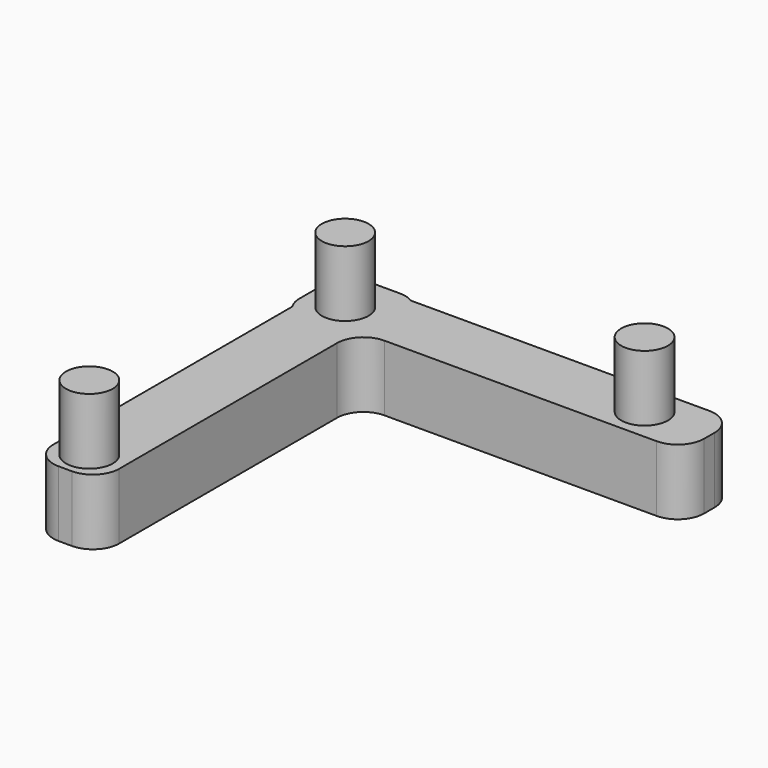
from build123d import *

# Parameters (mm, degrees)
F0_R         = 4.5120624022
F1_DEPTH     = 25.4
F0_W         = 0.7937453203
F0_H         = 12.7
F0_W_2       = 12.7
F0_H_2       = 0.7937453203
F2_DEPTH     = 12.7
F3_R         = 5.08
F4_T1_DEPTH  = 12.7
F4_T3_DEPTH  = 26.333067172
F4_T5_DEPTH  = 38.1
F4_T7_DEPTH  = 26.333067172
F4_T9_DEPTH  = 38.1
F4_T11_DEPTH = 26.333067172
F4_T13_DEPTH = 38.1
F4_T15_DEPTH = 26.333067172


# Not quite as in the source:
# - a fillet or chamfer that OpenCascade refuses, or shapes differently, is made with other operations: its cross-section is extruded or revolved along the edge and cut away or added


with BuildPart() as f1:
    # F0 (on Top) → F1 (new body)
    with BuildSketch(Plane.XY):
        with Locations((-30.9562546797, 29.4322539121)):
            Circle(F0_R)
    extrude(amount=F1_DEPTH)


with BuildPart() as f1b:
    # F0 (on Top) → F1, piece 2 (new body)
    with BuildSketch(Plane.XY):
        with Locations((25.6057605147, 30.9562546797)):
            Circle(F0_R)
    extrude(amount=F1_DEPTH)


with BuildPart() as f1c:
    # F0 (on Top) → F1, piece 3 (new body)
    with BuildSketch(Plane.XY):
        with Locations((-30.9562546797, -32.2909392416)):
            Circle(F0_R)
    extrude(amount=F1_DEPTH)


with BuildPart() as f2:
    # F0 (on Top) → F2 (new body)
    with BuildSketch(Plane.XY):
        Polygon((-37.3062546797, -38.1), (-24.6062546797, -38.1), (-24.6062546797, 24.6062546797), (38.1, 24.6062546797), (38.1, 37.3062546797), (-24.6062546797, 37.3062546797), (-37.3062546797, 37.3062546797), (-37.3062546797, 24.6062546797), align=None)
        with Locations((-30.9562546797, -32.2909392416)):
            Circle(F0_R, mode=Mode.SUBTRACT)
        with Locations((-30.9562546797, 29.4322539121)):
            Circle(F0_R, mode=Mode.SUBTRACT)
        with Locations((25.6057605147, 30.9562546797)):
            Circle(F0_R, mode=Mode.SUBTRACT)
        with Locations((-37.7031273399, 30.9562546797)):
            Rectangle(F0_W, F0_H)
        with Locations((-30.9562546797, 37.7031273399)):
            Rectangle(F0_W_2, F0_H_2)
    extrude(amount=F2_DEPTH)

    # F3
    f3_edges = [f2.edges().sort_by_distance(p)[0] for p in [
        (-37.306255, -38.1, 6.35),
    ]]
    fillet(f3_edges, radius=F3_R)

    # F4: fillet of radius 5.08 on 8 edges, made by hand

    # F4_s2 → F4_t1 (join)
    with BuildSketch(Plane.XY):
        with BuildLine():
            ThreePointArc((-24.6062546797, 19.5262546797), (-23.1183571281, 23.1183571281), (-19.5262546797, 24.6062546797))
            Line((-19.5262546797, 24.6062546797), (-24.6062546797, 24.6062546797))
            Line((-24.6062546797, 24.6062546797), (-24.6062546797, 19.5262546797))
        make_face()
    extrude(amount=F4_T1_DEPTH)

    # F4_s4 → F4_t3 (cut)
    with BuildSketch(Plane.XY.offset(-6.816533586)):
        with BuildLine():
            ThreePointArc((-37.3062546797, 24.6062546797), (-37.8975287684, 25.9129691341), (-38.1, 27.3328681141))
            Line((-38.1, 27.3328681141), (-38.1, 24.6062546797))
            Line((-38.1, 24.6062546797), (-37.3062546797, 24.6062546797))
        make_face()
    extrude(amount=F4_T3_DEPTH, mode=Mode.SUBTRACT)

    # F4_s6 → F4_t5 (cut)
    with BuildSketch(Plane.XY.offset(-12.7)):
        with BuildLine():
            ThreePointArc((-24.6062546797, -33.02), (-26.0941522313, -36.6121024484), (-29.6862546797, -38.1))
            Line((-29.6862546797, -38.1), (-24.6062546797, -38.1))
            Line((-24.6062546797, -38.1), (-24.6062546797, -33.02))
        make_face()
    extrude(amount=F4_T5_DEPTH, mode=Mode.SUBTRACT)

    # F4_s8 → F4_t7 (cut)
    with BuildSketch(Plane.XY.offset(-6.816533586)):
        with BuildLine():
            ThreePointArc((-38.1, 34.5796412453), (-37.8975287684, 35.9995402254), (-37.3062546797, 37.3062546797))
            Line((-37.3062546797, 37.3062546797), (-38.1, 37.3062546797))
            Line((-38.1, 37.3062546797), (-38.1, 34.5796412453))
        make_face()
    extrude(amount=F4_T7_DEPTH, mode=Mode.SUBTRACT)

    # F4_s10 → F4_t9 (cut)
    with BuildSketch(Plane.XY.offset(-12.7)):
        with BuildLine():
            ThreePointArc((38.1, 29.6862546797), (36.6121024484, 26.0941522313), (33.02, 24.6062546797))
            Line((33.02, 24.6062546797), (38.1, 24.6062546797))
            Line((38.1, 24.6062546797), (38.1, 29.6862546797))
        make_face()
    extrude(amount=F4_T9_DEPTH, mode=Mode.SUBTRACT)

    # F4_s12 → F4_t11 (cut)
    with BuildSketch(Plane.XY.offset(-6.816533586)):
        with BuildLine():
            ThreePointArc((-37.3062546797, 37.3062546797), (-35.9995402254, 37.8975287684), (-34.5796412453, 38.1))
            Line((-34.5796412453, 38.1), (-37.3062546797, 38.1))
            Line((-37.3062546797, 38.1), (-37.3062546797, 37.3062546797))
        make_face()
    extrude(amount=F4_T11_DEPTH, mode=Mode.SUBTRACT)

    # F4_s14 → F4_t13 (cut)
    with BuildSketch(Plane.XY.offset(-12.7)):
        with BuildLine():
            ThreePointArc((33.02, 37.3062546797), (36.6121024484, 35.8183571281), (38.1, 32.2262546797))
            Line((38.1, 32.2262546797), (38.1, 37.3062546797))
            Line((38.1, 37.3062546797), (33.02, 37.3062546797))
        make_face()
    extrude(amount=F4_T13_DEPTH, mode=Mode.SUBTRACT)

    # F4_s16 → F4_t15 (cut)
    with BuildSketch(Plane.XY.offset(-6.816533586)):
        with BuildLine():
            ThreePointArc((-27.3328681141, 38.1), (-25.9129691341, 37.8975287684), (-24.6062546797, 37.3062546797))
            Line((-24.6062546797, 37.3062546797), (-24.6062546797, 38.1))
            Line((-24.6062546797, 38.1), (-27.3328681141, 38.1))
        make_face()
    extrude(amount=F4_T15_DEPTH, mode=Mode.SUBTRACT)


solid = Compound([f1.part, f1b.part, f1c.part, f2.part])
